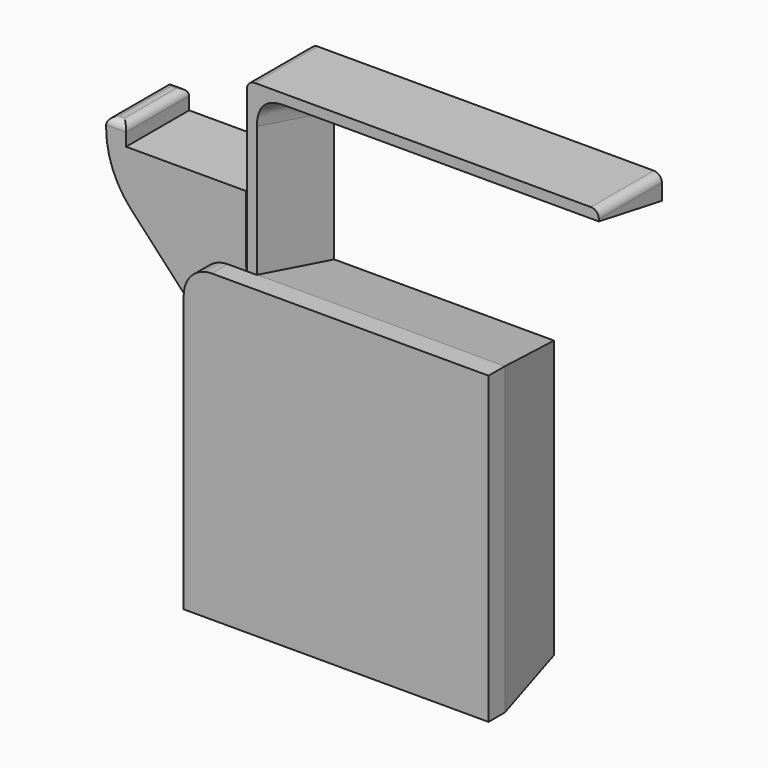
from build123d import *

# Parameters (mm, degrees)
F0_W        = 76.2
F0_H        = 76.2
F1_DEPTH    = 5
F2_R        = 7
F3_DEPTH    = 19.79
F4_C1_SIZE2 = 3.47364152
F4_C1_SIZE  = 19.7
F4_C2_SIZE2 = 19.7
F4_C2_SIZE  = 3.47364152
F4_C3_SIZE2 = 19.7
F4_C3_SIZE  = 3.47364152
F4_C4_SIZE2 = 19.7
F4_C4_SIZE  = 3.47364152
F5_T1_DEPTH = 88.2233868706
F7_DEPTH    = 19.7
F8_SIZE2    = 3.473632
F8_SIZE     = 19.69999
F9_T4_DEPTH = 54.2633149659
F11_DEPTH   = 19.7
F12_R       = 1.8106601718
F13_R       = 23.4632344254
F14_R       = 2
F15_R       = 2
F16_R       = 2


# Not quite as in the source:
# - a fillet or chamfer that OpenCascade refuses, or shapes differently, is made with other operations: its cross-section is extruded or revolved along the edge and cut away or added
# - a fillet or chamfer is up to 0.001 mm smaller than in the source, because OpenCascade refuses the exact size


with BuildPart() as f1:
    # F0 (on Front) → F1 (new body)
    with BuildSketch(Plane.XZ):
        Rectangle(F0_W, F0_H)
    extrude(amount=F1_DEPTH)

    # F2
    f2_edges = [f1.edges().sort_by_distance(p)[0] for p in [
        (-38.1, -2.5, 38.1),
    ]]
    fillet(f2_edges, radius=F2_R)

    # F0 (on Front) → F3 (join)
    with BuildSketch(Plane.XZ):
        Rectangle(F0_W, F0_H)
    extrude(amount=-F3_DEPTH)

    # F4: chamfer of 19.7 x 3.47364152 on 4 edges, made by hand

    # F4_c1
    f4_c1_edges = [f1.edges().sort_by_distance(p)[0] for p in [
        (0, 19.79, 38.1),
    ]]
    f4_c1_side = f1.faces().sort_by_distance((0, 19.7205271696, 38.1))[0]
    chamfer(f4_c1_edges, length=F4_C1_SIZE, length2=F4_C1_SIZE2, reference=f4_c1_side)

    # F4_c2
    f4_c2_edges = [f1.edges().sort_by_distance(p)[0] for p in [
        (0, 19.79, -38.1),
    ]]
    f4_c2_side = f1.faces().sort_by_distance((0, 19.79, -38.0305271696))[0]
    chamfer(f4_c2_edges, length=F4_C2_SIZE, length2=F4_C2_SIZE2, reference=f4_c2_side)

    # F4_c3
    f4_c3_edges = [f1.edges().sort_by_distance(p)[0] for p in [
        (38.1, 19.79, 0),
    ]]
    f4_c3_side = f1.faces().sort_by_distance((38.0305271696, 19.79, 0))[0]
    chamfer(f4_c3_edges, length=F4_C3_SIZE, length2=F4_C3_SIZE2, reference=f4_c3_side)

    # F4_c4
    f4_c4_edges = [f1.edges().sort_by_distance(p)[0] for p in [
        (-38.1, 19.79, 0),
    ]]
    f4_c4_side = f1.faces().sort_by_distance((-38.0305271696, 19.79, 0))[0]
    chamfer(f4_c4_edges, length=F4_C4_SIZE, length2=F4_C4_SIZE2, reference=f4_c4_side)

    # F5: fillet of radius 7 on 1 edges, made by hand

    # F5_s2 → F5_t1 (cut)
    with BuildSketch(Plane(origin=(4.1632046596, 23.6107068972, -4.1632046596), x_dir=(0.984807753, -0.1736481777, 0), z_dir=(-0.1710878697, -0.9702875252, 0.1710878697))):
        with BuildLine():
            ThreePointArc((-37.5368037258, 29.629479716), (-35.560623527, 34.5040293983), (-30.747879553, 36.6262966348))
            Line((-30.747879553, 36.6262966348), (-37.5368037258, 36.4214923928))
            Line((-37.5368037258, 36.4214923928), (-37.5368037258, 29.629479716))
        make_face()
    extrude(amount=F5_T1_DEPTH, mode=Mode.SUBTRACT)


with BuildPart() as f7:
    # F6 (on Front) → F7 (new body)
    with BuildSketch(Plane.XZ):
        Polygon((-26.3288263232, 80.1959456988), (-26.3288263232, -7.8040543012), (-20.3288263232, -7.8040543012), (-20.3288263232, 74.1959456988), (61.6711736768, 74.1959456988), (61.6711736768, 80.1959456988), align=None)
    extrude(amount=-F7_DEPTH)

    # F8 (size 19.7 and 3.47364152 in the source; OpenCascade refuses exactly that, so slightly less here)
    f8_edges = [f7.edges().sort_by_distance(p)[0] for p in [
        (-20.328826, 0, 33.195946),
        (20.671174, 0, 74.195946),
    ]]
    chamfer(f8_edges, length=F8_SIZE, length2=F8_SIZE2)

    # F9: fillet of radius 7 on 1 edges, made by hand


with BuildPart() as f9_tool2:
    # F9_s3 → F9_t4 (new body)
    with BuildSketch(Plane(origin=(3.4085222403, 19.330733379, -3.4085222403), x_dir=(0.9848078193, -0.1736478016, 0), z_dir=(-0.1710875101, -0.9702876521, 0.1710875101))):
        with BuildLine():
            add(Edge.make_bspline(
                [(-23.4408470757, 69.0252446825), (-23.4408470757, 75.8172582472), (-16.6519219887, 76.0220616289)],
                knots=[0, 0, 0, 1, 1, 1], degree=2, weights=[1, 1, 1]))
            Line((-16.6519219887, 76.0220616289), (-16.656143487, 76.1619979678))
            Line((-16.656143487, 76.1619979678), (-23.5808470757, 75.9530985184))
            Line((-23.5808470757, 75.9530985184), (-23.5808470757, 69.0252446825))
            Line((-23.5808470757, 69.0252446825), (-23.4408470757, 69.0252446825))
        make_face()
    extrude(amount=F9_T4_DEPTH)

    split(bisect_by=Plane.XZ.offset(-19.7), keep=Keep.TOP)

    split(bisect_by=Plane.XZ, keep=Keep.BOTTOM)


with BuildPart() as f7_1:
    add(f7.part)

    # F9_t1: union F9_tool2
    add(f9_tool2.part)

    # F14
    f14_edges = [f7_1.edges().sort_by_distance(p)[0] for p in [
        (-26.328826, 9.85, 80.195946),
    ]]
    fillet(f14_edges, radius=F14_R)

    # F15
    f15_edges = [f7_1.edges().sort_by_distance(p)[0] for p in [
        (-26.328826, 9.85, -7.804054),
    ]]
    fillet(f15_edges, radius=F15_R)

    # F16
    f16_edges = [f7_1.edges().sort_by_distance(p)[0] for p in [
        (61.671174, 9.85, 80.195946),
    ]]
    fillet(f16_edges, radius=F16_R)


with BuildPart() as f11:
    # F10 (on Front) → F11 (new body)
    with BuildSketch(Plane.XZ):
        Polygon((-26.4252573252, 11.3248322159), (-26.4958144724, 55.6931681931), (-56.4958144724, 55.6931681931), (-56.4958144724, 60.6931681931), (-61.4958144724, 60.6931681931), (-61.4958144724, 49.005292356), align=None)
    extrude(amount=-F11_DEPTH)

    # F12
    f12_edges = [f11.edges().sort_by_distance(p)[0] for p in [
        (-56.495814, 9.85, 60.693168),
        (-61.495814, 9.85, 60.693168),
        (-58.995814, 0, 60.693168),
        (-58.995814, 19.7, 60.693168),
    ]]
    fillet(f12_edges, radius=F12_R)

    # F13
    f13_edges = [f11.edges().sort_by_distance(p)[0] for p in [
        (-61.495814, 9.85, 49.005292),
    ]]
    fillet(f13_edges, radius=F13_R)


solid = Compound([f1.part, f7_1.part, f11.part])
